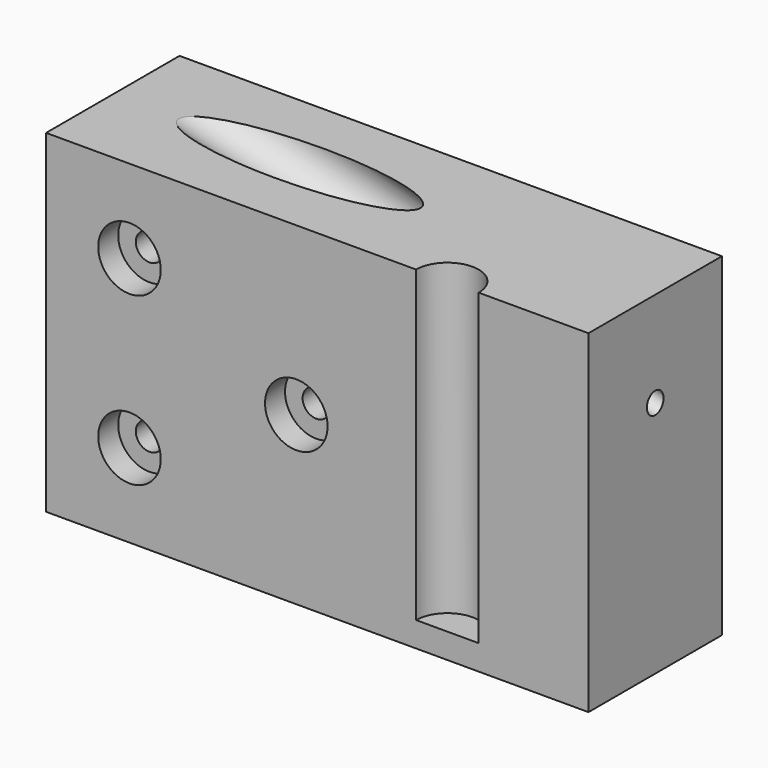
from build123d import *

# Parameters (mm, degrees)
F0_W            = 76.2
F0_H            = 50.8
F1_DEPTH        = 25.4
F3_DEPTH        = 25.401
F5_D            = 9.525
F7_DEPTH        = 25.401
F9_DEPTH        = 25.401
F11_DEPTH       = 25.4
F13_D           = 3.175
F15_DEPTH       = 46.99
F17_D           = 4.1656
F17_CBORE_D     = 9.525
F17_CBORE_DEPTH = 3.81


with BuildPart() as f1:
    # F0 (on Front) → F1 (new body)
    with BuildSketch(Plane.XZ):
        Rectangle(F0_W, F0_H)
    extrude(amount=F1_DEPTH)

    # F2 (on face) → F3 (cut, through all)
    with BuildSketch(Plane.XZ.offset(25.4)):
        Polygon((38.1, -25.4), (38.1, 25.4), (24.4881810245, -25.4), align=None)
    extrude(amount=-F3_DEPTH, mode=Mode.SUBTRACT)

    # F5 (through all)
    with Locations(Plane(origin=(29.1977839421, 0, -7.8235226281), x_dir=(0, 1, 0), z_dir=(0.9659258263, 0, -0.2588190451))):
        with Locations((-12.7, 22.0410656184)):
            Hole(F5_D / 2)

    # F6 (on face) → F7 (cut, through all)
    with BuildSketch(Plane(origin=(0, 0, 0), x_dir=(-1, 0, 0), z_dir=(0, 1, 0))):
        Polygon((-24.4881810245, 25.4), (-38.1, 25.4), (-24.4881810245, -25.4), align=None)
    extrude(amount=-F7_DEPTH, mode=Mode.SUBTRACT)

    # F8 (on face) → F9 (cut, through all)
    with BuildSketch(Plane.XZ.offset(25.4)):
        Polygon((24.4881810245, -25.4), (24.4881810245, 25.4), (10.876362049, -25.4), align=None)
    extrude(amount=-F9_DEPTH, mode=Mode.SUBTRACT)

    # F10 (on face) → F11 (join)
    with BuildSketch(Plane.XZ.offset(25.4)):
        Polygon((44.4944761693, 25.4), (24.4881810245, 25.4), (10.876362049, -25.4), (44.4944761693, -25.4), align=None)
    extrude(amount=-F11_DEPTH)

    # F13 (through all)
    with Locations(Plane(origin=(16.4977839421, 0, -4.4205678842), x_dir=(0, -1, 0), z_dir=(-0.9659258263, 0, 0.2588190451))):
        with Locations((12.7, 22.0410656184)):
            Hole(F13_D / 2)

    # F14 (on face) → F15 (cut)
    with BuildSketch(Plane.XY.offset(25.4)):
        with BuildLine():
            ThreePointArc((27.7756870478, -25.4), (23.0131870478, -20.6375), (18.2506870478, -25.4))
            Line((18.2506870478, -25.4), (27.7756870478, -25.4))
        make_face()
    extrude(amount=-F15_DEPTH, mode=Mode.SUBTRACT)

    # F17 (through all)
    with Locations(Plane.XZ.offset(25.4)):
        with Locations((-25.4, -12.7), (-25.4, 12.7), (0, 0)):
            CounterBoreHole(F17_D / 2, F17_CBORE_D / 2, F17_CBORE_DEPTH)


solid = f1.part
